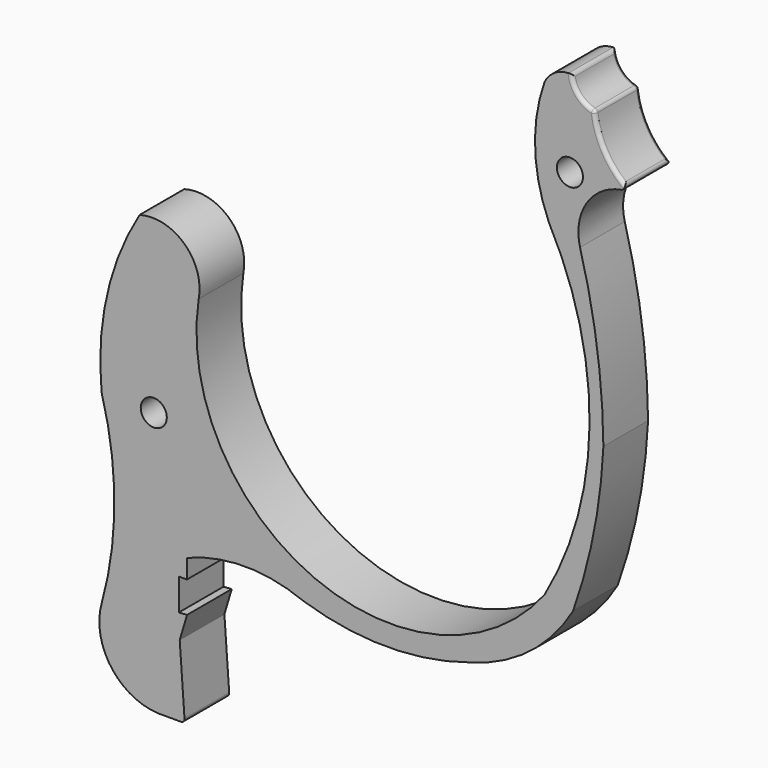
from build123d import *

# Parameters (mm, degrees)
F1_DEPTH       = 3.81
F2_R           = 0.254
F3_D           = 1.778
F3_CSINK_D     = 3.175
F3_CSINK_ANGLE = 82


# Not quite as in the source:
# - a feature names something its author has since deleted; it is built from what else it names


with BuildPart() as f1:
    # F0 (on Front) → F1 (new body)
    with BuildSketch(Plane.XZ):
        with BuildLine():
            ThreePointArc((-15.3976073489, 30.0757028162), (-12.6205023663, 18.8138288447), (-15.6854130328, 7.6268524863))
            ThreePointArc((-15.6854130328, 7.6268524863), (-31.3905262472, 3.5144175537), (-39.2854884267, 17.7000537515))
            ThreePointArc((-39.2854884267, 17.7000537515), (-40.2547680717, 20.6965618199), (-43.3147661388, 21.4415285736))
            ThreePointArc((-43.3147661388, 21.4415285736), (-45.5440273695, 15.8957464039), (-45.905020088, 9.9295927212))
            ThreePointArc((-45.905020088, 9.9295927212), (-45.0345404234, 3.597348812), (-45.905020088, -2.7348950971))
            ThreePointArc((-45.905020088, -2.7348950971), (-45.1259294206, -6.5201466433), (-41.5899753571, -8.0796787515))
            Line((-41.5899753571, -8.0796787515), (-40.2320445972, -8.0796787515))
            Line((-40.2320445972, -8.0796787515), (-40.5776619182, -3.1953468446))
            Line((-40.5776619182, -3.1953468446), (-40.0765932374, -1.5246287875))
            Line((-40.0765932374, -1.5246287875), (-40.6392291188, -1.5644411324))
            Line((-40.6392291188, -1.5644411324), (-40.6392291188, 0.5960793933))
            Line((-40.6392291188, 0.5960793933), (-40.0844532998, 0.5960793933))
            Line((-40.0844532998, 0.5960793933), (-40.0844532998, 1.8968694892))
            ThreePointArc((-40.0844532998, 1.8968694892), (-36.1157211919, 2.6708049351), (-32.1480344873, 1.8915278128))
            ThreePointArc((-32.1480344873, 1.8915278128), (-26.4720596319, 0.9912977201), (-20.7960847765, 1.8915278128))
            ThreePointArc((-20.7960847765, 1.8915278128), (-16.7308465178, 3.8739299722), (-13.7448431924, 7.2709675878))
            ThreePointArc((-13.7448431924, 7.2709675878), (-12.3233048625, 12.470180408), (-11.6768007285, 17.821312772))
            ThreePointArc((-11.6768007285, 17.821312772), (-12.1024444853, 23.5936908911), (-13.2695324719, 29.2628555023))
            ThreePointArc((-13.2695324719, 29.2628555023), (-12.6323011565, 32.3319998397), (-9.8052835092, 33.6861349642))
            ThreePointArc((-9.8052835092, 33.6861349642), (-11.5106118889, 35.4421925399), (-12.2696207836, 37.7693772316))
            ThreePointArc((-12.2696207836, 37.7693772316), (-13.3462306374, 38.3418830024), (-13.8277616352, 39.4621416926))
            ThreePointArc((-13.8277616352, 39.4621416926), (-14.9168802382, 39.2283992754), (-15.6854130328, 38.4220667183))
            ThreePointArc((-15.6854130328, 38.4220667183), (-16.3374101507, 34.221439938), (-15.3976073489, 30.0757028162))
        make_face()
    extrude(amount=F1_DEPTH)

    # F2
    f2_edges = [f1.edges().sort_by_distance(p)[0] for p in [
        (-45.90502, -1.905, -2.734895),
        (-13.827762, -1.905, 39.462142),
        (-12.269621, -1.905, 37.769377),
        (-13.346231, 0, 38.341883),
        (-13.346231, -3.81, 38.341883),
        (-11.510612, -3.81, 35.442193),
        (-11.510612, 0, 35.442193),
        (-9.805284, -1.905, 33.686135),
        (-40.232045, -1.905, -8.079679),
    ]]
    fillet(f2_edges, radius=F2_R)

    # F3 (through all)
    with Locations(Plane(origin=(0, 0, 0), x_dir=(1, 0, 0), z_dir=(0, 1, 0))):
        with Locations((-42.347650975, -9.8781445995), (-13.9591796324, -33.550273627)):
            CounterSinkHole(F3_D / 2, F3_CSINK_D / 2, counter_sink_angle=F3_CSINK_ANGLE)


solid = f1.part
